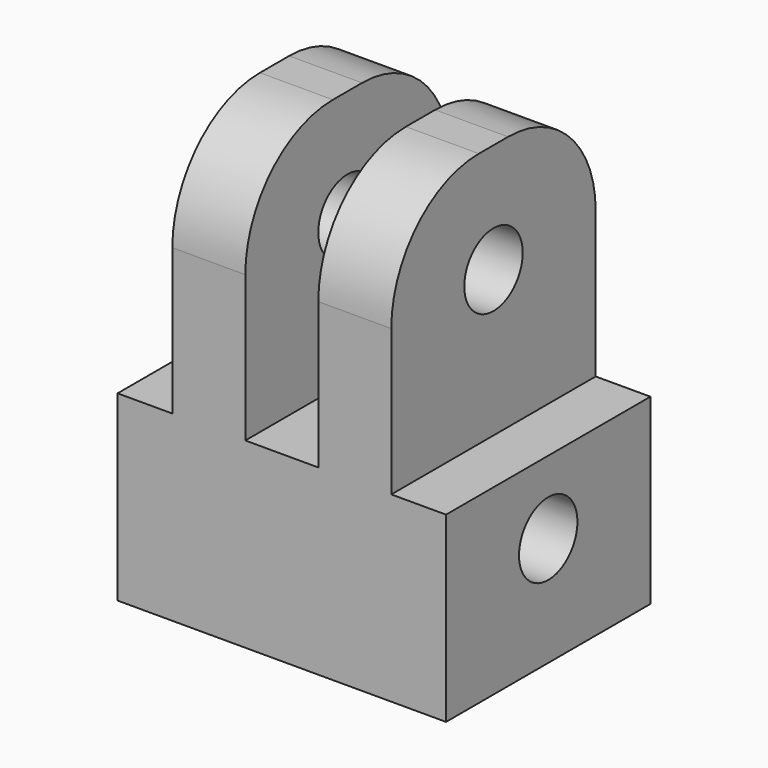
from build123d import *

# Parameters (mm, degrees)
F0_W     = 114.3
F0_H     = 88.9
F1_DEPTH = 152.4
F3_R     = 38.1
F4_R     = 12.7
F5_DEPTH = 114.301
F6_R     = 6.35
F7_DEPTH = 38.1
F2_W     = 19.05
F2_H     = 88.9
F2_W_2   = 25.4
F8_DEPTH = 88.901


with BuildPart() as f1:
    # F0 (on Top) → F1 (new body)
    with BuildSketch(Plane.XY):
        Rectangle(F0_W, F0_H)
    extrude(amount=F1_DEPTH)

    # F3
    f3_edges = [f1.edges().sort_by_distance(p)[0] for p in [
        (0, -44.45, 152.4),
        (0, 44.45, 152.4),
    ]]
    fillet(f3_edges, radius=F3_R)

    # F4 (on face) → F5 (cut, through all)
    with BuildSketch(Plane(origin=(-57.15, 0, 0), x_dir=(0, -1, 0), z_dir=(-1, 0, 0))):
        with Locations((0, 38.1)):
            Circle(F4_R)
        with Locations((0, 114.3)):
            Circle(F4_R)
    extrude(amount=-F5_DEPTH, mode=Mode.SUBTRACT)

    # F6 (on face) → F7 (cut)
    with BuildSketch(Plane(origin=(0, 0, 0), x_dir=(1, 0, 0), z_dir=(0, 0, -1))):
        Circle(F6_R)
    extrude(amount=-F7_DEPTH, mode=Mode.SUBTRACT)

    # F2 (on face) → F8 (cut, through all)
    with BuildSketch(Plane.XZ.offset(44.45)):
        with Locations((-47.625, 107.95)):
            Rectangle(F2_W, F2_H)
        with Locations((0, 107.95)):
            Rectangle(F2_W_2, F2_H)
        with Locations((47.625, 107.95)):
            Rectangle(F2_W, F2_H)
    extrude(amount=-F8_DEPTH, mode=Mode.SUBTRACT)


solid = f1.part
